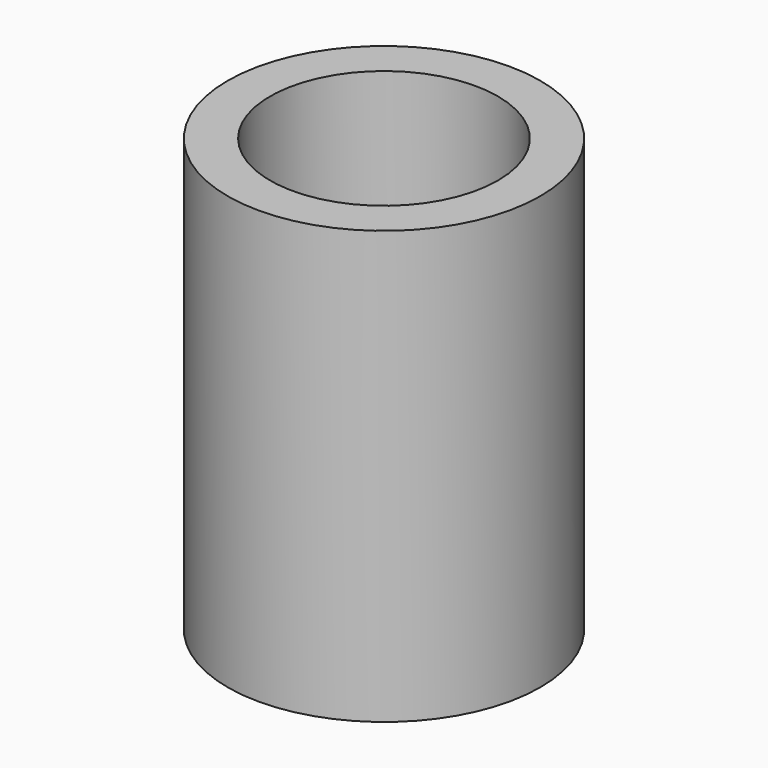
from build123d import *

# Parameters (mm, degrees)
F0_R     = 74.2865291694
F1_DEPTH = 151.892
F2_DEPTH = 53.594
F3_R     = 54.1549709352
F4_DEPTH = 195.58
F5_DEPTH = 92.202


# Not quite as in the source:
# - a feature names something its author has since deleted; it is built from what else it names


with BuildPart() as f1:
    # F0 (on Top) → F1 (new body)
    with BuildSketch(Plane.XY):
        Circle(F0_R)
    extrude(amount=F1_DEPTH)

    # F2 (add): a face of the model
    f2_faces = [f1.faces().sort_by_distance(p)[0] for p in [
        (0, 0, 151.892),
    ]]
    extrude(f2_faces, amount=F2_DEPTH)

    # F3 (on face) → F4 (cut)
    with BuildSketch(Plane.XY.offset(205.486)):
        Circle(F3_R)
    extrude(amount=-F4_DEPTH, mode=Mode.SUBTRACT)

    # F5 (cut): a face of the model
    f5_faces = [f1.faces().sort_by_distance(p)[0] for p in [
        (0, 0, 9.906),
    ]]
    extrude(f5_faces, amount=-F5_DEPTH, mode=Mode.SUBTRACT)


solid = f1.part
